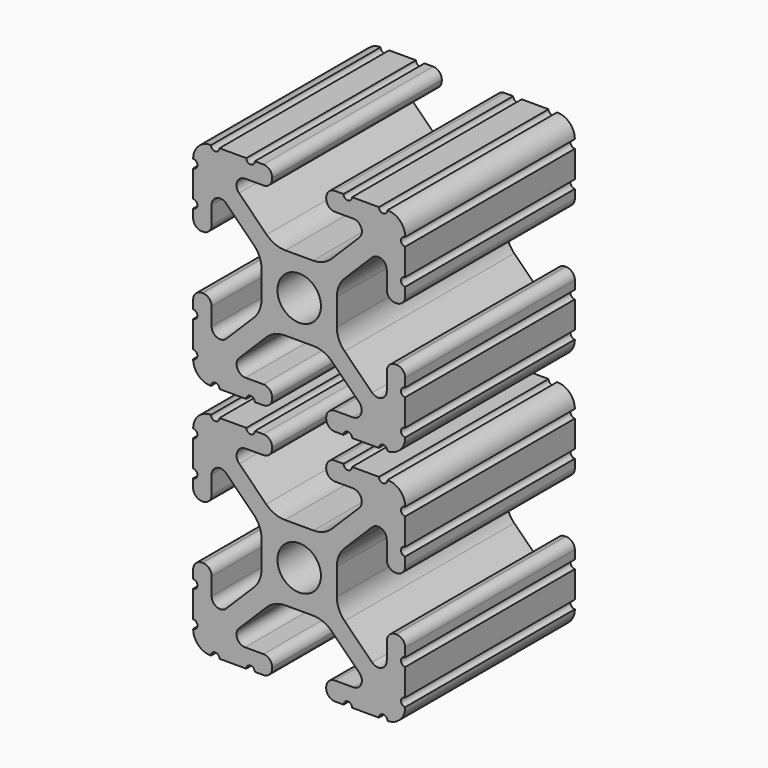
from build123d import *

# Parameters (mm, degrees)
F0_R     = 2.5625
F2_DEPTH = 12.5


# Not quite as in the source:
# - ends of sketch curves that miss each other by under 0.0002 mm in the source are joined


with BuildPart() as f2:
    # F0 (on Front) → F2 (new body, symmetric)
    with BuildSketch(Plane.XZ):
        with BuildLine():
            ThreePointArc((-3.8900202791, -5.3382797295), (-2.8768958758, -4.6623321828), (-1.682325, -4.425))
            Line((-1.682325, -4.425), (1.682325, -4.425))
            ThreePointArc((1.682325, -4.425), (2.8768958758, -4.6623321828), (3.8900202791, -5.3382797295))
            Line((3.8900202791, -5.3382797295), (7.066575, -8.50905))
            ThreePointArc((7.066575, -8.50905), (7.2979716135, -9.6681190856), (6.315375, -10.325))
            Line((6.315375, -10.325), (4.22, -10.325))
            ThreePointArc((4.22, -10.325), (3.4899122484, -10.6274122484), (3.1875, -11.3575))
            Line((3.1875, -11.3575), (3.1875, -11.4675))
            ThreePointArc((3.1875, -11.4675), (3.4899122484, -12.1975877516), (4.22, -12.5))
            Line((4.22, -12.5), (5.2334, -12.5))
            ThreePointArc((5.2334, -12.5), (5.7334, -12), (6.2334, -12.5))
            Line((6.2334, -12.5), (9.40005, -12.5))
            ThreePointArc((9.40005, -12.5), (9.899975, -12.0000000056), (10.4000499775, -12.49985))
            ThreePointArc((10.4000499775, -12.49985), (11.8922642472, -11.8922288945), (12.4998493922, -10.4000000073))
            ThreePointArc((12.4998493922, -10.4000000073), (12.0000000056, -9.899925), (12.5, -9.4))
            Line((12.5, -9.4), (12.5, -6.23335))
            ThreePointArc((12.5, -6.23335), (12, -5.73335), (12.5, -5.23335))
            Line((12.5, -5.23335), (12.5, -4.21995))
            ThreePointArc((12.5, -4.21995), (12.1975877516, -3.4898622484), (11.4675, -3.18745))
            Line((11.4675, -3.18745), (11.3575, -3.18745))
            ThreePointArc((11.3575, -3.18745), (10.6274122484, -3.4898622484), (10.325, -4.21995))
            Line((10.325, -4.21995), (10.325, -6.301275))
            ThreePointArc((10.325, -6.301275), (9.7012847872, -7.2353050667), (8.5995439137, -7.0171311001))
            Line((8.5995439137, -7.0171311001), (5.355325, -3.780325))
            ThreePointArc((5.355325, -3.780325), (4.6760601946, -2.7656350724), (4.4375, -1.5681))
            Line((4.4375, -1.5681), (4.4375, 1.5681))
            ThreePointArc((4.4375, 1.5681), (4.6760601946, 2.7656350724), (5.3553177597, 3.7803322568))
            Line((5.3553177597, 3.7803322568), (8.59955, 7.017125))
            ThreePointArc((8.59955, 7.017125), (9.7012847872, 7.2353050667), (10.325, 6.301275))
            Line((10.325, 6.301275), (10.325, 4.21995))
            ThreePointArc((10.325, 4.21995), (10.6274122484, 3.4898622484), (11.3575, 3.18745))
            Line((11.3575, 3.18745), (11.4675, 3.18745))
            ThreePointArc((11.4675, 3.18745), (12.1975877516, 3.4898622484), (12.5, 4.21995))
            Line((12.5, 4.21995), (12.5, 5.23335))
            ThreePointArc((12.5, 5.23335), (12, 5.73335), (12.5, 6.23335))
            Line((12.5, 6.23335), (12.5, 9.4))
            ThreePointArc((12.5, 9.4), (12.0000000056, 9.899925), (12.49985, 10.3999999775))
            ThreePointArc((12.49985, 10.3999999775), (11.8922642472, 11.8922288945), (10.40005, 12.499849994))
            ThreePointArc((10.40005, 12.499849994), (9.899975, 12.0000000056), (9.40005, 12.5))
            Line((9.40005, 12.5), (6.2334, 12.5))
            ThreePointArc((6.2334, 12.5), (5.7334, 12), (5.2334, 12.5))
            Line((5.2334, 12.5), (4.22, 12.5))
            ThreePointArc((4.22, 12.5), (3.4899122484, 12.1975877516), (3.1875, 11.4675))
            Line((3.1875, 11.4675), (3.1875, 11.3575))
            ThreePointArc((3.1875, 11.3575), (3.4899122484, 10.6274122484), (4.22, 10.325))
            Line((4.22, 10.325), (6.3748, 10.325))
            ThreePointArc((6.3748, 10.325), (7.3151859964, 9.696264211), (7.0935440721, 8.5869809415))
            Line((7.0935440721, 8.5869809415), (3.836875, 5.337775))
            ThreePointArc((3.836875, 5.337775), (2.8239359895, 4.6621936697), (1.6297, 4.425))
            Line((1.6297, 4.425), (-1.6297, 4.425))
            ThreePointArc((-1.6297, 4.425), (-2.8239359895, 4.6621936697), (-3.8368822403, 5.3377677432))
            Line((-3.8368822403, 5.3377677432), (-7.09355, 8.586975))
            ThreePointArc((-7.09355, 8.586975), (-7.3151859964, 9.696264211), (-6.3748, 10.325))
            Line((-6.3748, 10.325), (-4.22, 10.325))
            ThreePointArc((-4.22, 10.325), (-3.4899122484, 10.6274122484), (-3.1875, 11.3575))
            Line((-3.1875, 11.3575), (-3.1875, 11.4675))
            ThreePointArc((-3.1875, 11.4675), (-3.4899122484, 12.1975877516), (-4.22, 12.5))
            Line((-4.22, 12.5), (-5.2334, 12.5))
            ThreePointArc((-5.2334, 12.5), (-5.7334, 12), (-6.2334, 12.5))
            Line((-6.2334, 12.5), (-9.40005, 12.5))
            ThreePointArc((-9.40005, 12.5), (-9.899975, 12.0000000056), (-10.4000499775, 12.49985))
            ThreePointArc((-10.4000499775, 12.49985), (-11.8922642472, 11.8922288945), (-12.4998493922, 10.4000000073))
            ThreePointArc((-12.4998493922, 10.4000000073), (-12.0000000056, 9.899925), (-12.5, 9.4))
            Line((-12.5, 9.4), (-12.5, 6.23335))
            ThreePointArc((-12.5, 6.23335), (-12, 5.73335), (-12.5, 5.23335))
            Line((-12.5, 5.23335), (-12.5, 4.21995))
            ThreePointArc((-12.5, 4.21995), (-12.1975877516, 3.4898622484), (-11.4675, 3.18745))
            Line((-11.4675, 3.18745), (-11.3575, 3.18745))
            ThreePointArc((-11.3575, 3.18745), (-10.6274122484, 3.4898622484), (-10.325, 4.21995))
            Line((-10.325, 4.21995), (-10.325, 6.301275))
            ThreePointArc((-10.325, 6.301275), (-9.7012847872, 7.2353050667), (-8.5995439137, 7.0171311001))
            Line((-8.5995439137, 7.0171311001), (-5.355325, 3.780325))
            ThreePointArc((-5.355325, 3.780325), (-4.6760601946, 2.7656350724), (-4.4375, 1.5681))
            Line((-4.4375, 1.5681), (-4.4375, -1.5681))
            ThreePointArc((-4.4375, -1.5681), (-4.6760601946, -2.7656350724), (-5.3553177597, -3.7803322568))
            Line((-5.3553177597, -3.7803322568), (-8.59955, -7.017125))
            ThreePointArc((-8.59955, -7.017125), (-9.7012847872, -7.2353050667), (-10.325, -6.301275))
            Line((-10.325, -6.301275), (-10.325, -4.21995))
            ThreePointArc((-10.325, -4.21995), (-10.6274122484, -3.4898622484), (-11.3575, -3.18745))
            Line((-11.3575, -3.18745), (-11.4675, -3.18745))
            ThreePointArc((-11.4675, -3.18745), (-12.1975877516, -3.4898622484), (-12.5, -4.21995))
            Line((-12.5, -4.21995), (-12.5, -5.23335))
            ThreePointArc((-12.5, -5.23335), (-12, -5.73335), (-12.5, -6.23335))
            Line((-12.5, -6.23335), (-12.5, -9.4))
            ThreePointArc((-12.5, -9.4), (-12.0000000056, -9.899925), (-12.49985, -10.3999999775))
            ThreePointArc((-12.49985, -10.3999999775), (-11.8922642472, -11.8922288945), (-10.40005, -12.499849994))
            ThreePointArc((-10.40005, -12.499849994), (-9.899975, -12.0000000056), (-9.40005, -12.5))
            Line((-9.40005, -12.5), (-6.2334, -12.5))
            ThreePointArc((-6.2334, -12.5), (-5.7334, -12), (-5.2334, -12.5))
            Line((-5.2334, -12.5), (-4.22, -12.5))
            ThreePointArc((-4.22, -12.5), (-3.4899122484, -12.1975877516), (-3.1875, -11.4675))
            Line((-3.1875, -11.4675), (-3.1875, -11.3575))
            ThreePointArc((-3.1875, -11.3575), (-3.4899122484, -10.6274122484), (-4.22, -10.325))
            Line((-4.22, -10.325), (-6.315375, -10.325))
            ThreePointArc((-6.315375, -10.325), (-7.2979716135, -9.6681190856), (-7.0665766684, -8.5090483285))
            Line((-7.0665766684, -8.5090483285), (-3.8900202791, -5.3382797295))
        make_face()
        Circle(F0_R, mode=Mode.SUBTRACT)
    extrude(amount=F2_DEPTH, both=True)


with BuildPart() as f2_1:
    # F3: moved
    add(f2.part.moved(Location((0, 0, 14))))


with BuildPart() as f4_1:
    # F4: instance of F2
    add(f2_1.part.mirror(Plane.XY))


solid = Compound([f2_1.part, f4_1.part])
